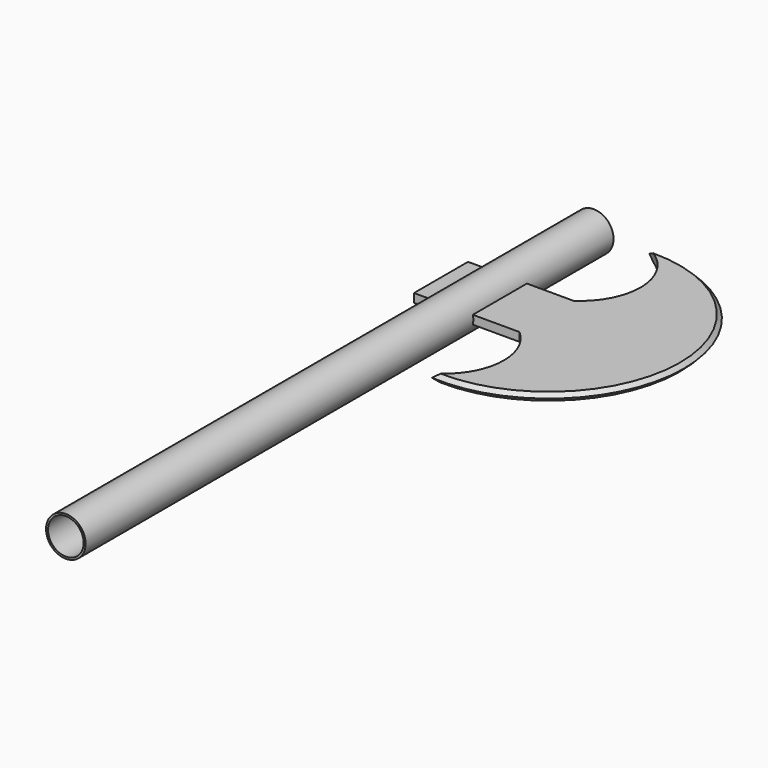
from build123d import *

# Parameters (mm, degrees)
F0_R          = 15
F0_R_2        = 13.5
F1_DEPTH      = 500
F2_W          = 51.2043386698
F2_H          = 6.5736337565
F3_DEPTH      = 50
F3_DEPTH_BACK = 30
F5_DEPTH      = 6
F6_T2_ANGLE   = 204.9841859294
F6_T4_ANGLE   = 204.9841859294


# Not quite as in the source:
# - a fillet or chamfer that OpenCascade refuses, or shapes differently, is made with other operations: its cross-section is extruded or revolved along the edge and cut away or added


with BuildPart() as f1:
    # F0 (on Front) → F1 (new body)
    with BuildSketch(Plane.XZ):
        Circle(F0_R)
        Circle(F0_R_2, mode=Mode.SUBTRACT)
    extrude(amount=F1_DEPTH)


with BuildPart() as f3:
    # F2 (on Right) → F3 (new body, two sides)
    with BuildSketch(Plane.YZ) as f3_sk:
        with Locations((-107.200242579, 0)):
            Rectangle(F2_W, F2_H)
    extrude(amount=F3_DEPTH)
    extrude(f3_sk.sketch, amount=-F3_DEPTH_BACK)

    # F4 (on face) → F5 (join)
    with BuildSketch(Plane.XY.offset(3.2868168782)):
        with BuildLine():
            ThreePointArc((39.1590334475, 0), (69.8835121208, -37.437195382), (50, -81.5980732441))
            Line((50, -81.5980732441), (50, -132.8024119139))
            ThreePointArc((50, -132.8024119139), (64.9970619773, -173.4303852551), (39.1590334475, -208.1858217716))
            ThreePointArc((39.1590334475, -208.1858217716), (153.6228645246, -104.0929108858), (39.1590334475, 0))
        make_face()
    extrude(amount=-F5_DEPTH)

    # F6: chamfer of 5 on 2 edges, made by hand

    # F6_s1 → F6_t2 (revolve, cut)
    with BuildSketch(Plane(origin=(68.7474753005, -15.2309949436, 0), x_dir=(0, 0, 1), z_dir=(-0.9763258673, 0.2163048793, 0))):
        Polygon((2.2868168782, -195.5793924312), (-2.7131831218, -190.5793924312), (-2.7131831218, -195.5793924312), align=None)
    revolve(axis=Axis((49.0601284346, -104.0929108858, -2.7131831218), (0, 0, 1)), revolution_arc=F6_T2_ANGLE, mode=Mode.SUBTRACT)

    # F6_s3 → F6_t4 (revolve, cut)
    with BuildSketch(Plane(origin=(68.7474753005, -15.2309949436, 0), x_dir=(0, 0, 1), z_dir=(-0.9763258673, 0.2163048793, 0))):
        Polygon((3.2868168782, -190.5793924312), (-1.7131831218, -195.5793924312), (3.2868168782, -195.5793924312), align=None)
    revolve(axis=Axis((49.0601284346, -104.0929108858, 3.2868168782), (0, 0, 1)), revolution_arc=F6_T4_ANGLE, mode=Mode.SUBTRACT)


solid = Compound([f1.part, f3.part])
